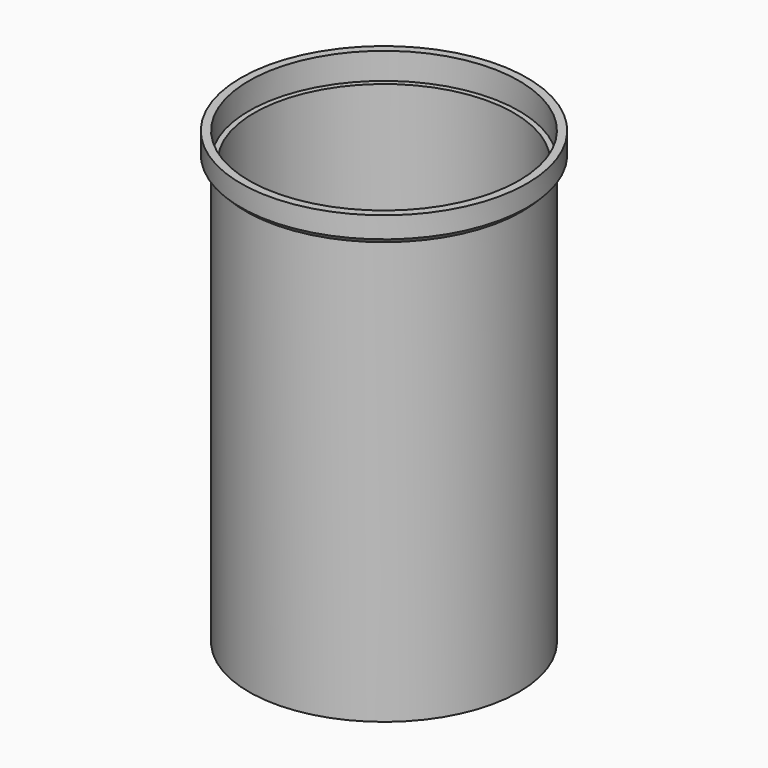
from build123d import *

# Parameters (mm, degrees)
F0_R          = 32.385
F1_DEPTH      = 101.6
F2_R          = 31.115
F3_DEPTH      = 99.06
F4_R          = 3.0308866689
F5_DEPTH      = 88.9
F5_DEPTH_BACK = 6.35
F6_R          = 34.3131351295
F6_R_2        = 32.385
F7_DEPTH      = 6.35
F8_SIZE       = 1.27


with BuildPart() as f1:
    # F0 (on Top) → F1 (new body)
    with BuildSketch(Plane.XY):
        Circle(F0_R)
    extrude(amount=F1_DEPTH)

    # F2 (on face) → F3 (cut)
    with BuildSketch(Plane.XY.offset(101.6)):
        Circle(F2_R)
    extrude(amount=-F3_DEPTH, mode=Mode.SUBTRACT)

    # F4 (on face) → F5 (cut, two sides)
    with BuildSketch(Plane.XY) as f5_sk:
        with Locations((-26.1913072318, 0)):
            Circle(F4_R)
        with Locations((-12.9833072318, 0)):
            Circle(F4_R)
        with Locations((0.2246927682, 0)):
            Circle(F4_R)
        with Locations((-21.1892126554, -15.3948641291)):
            Circle(F4_R)
        with Locations((-8.0935590395, -24.9094134131)):
            Circle(F4_R)
        with Locations((8.0935590395, -24.9094134131)):
            Circle(F4_R)
        with Locations((21.1892126554, -15.3948641291)):
            Circle(F4_R)
        with Locations((26.1913072318, 0)):
            Circle(F4_R)
        with Locations((21.1892126554, 15.3948641291)):
            Circle(F4_R)
        with Locations((8.0935590395, 24.9094134131)):
            Circle(F4_R)
        with Locations((-8.0935590395, 24.9094134131)):
            Circle(F4_R)
        with Locations((-21.1892126554, 15.3948641291)):
            Circle(F4_R)
        with Locations((-8.0949596534, -10.1507583404)):
            Circle(F4_R)
        with Locations((2.8890576511, -12.6577886127)):
            Circle(F4_R)
        with Locations((11.6975556182, -5.6332458878)):
            Circle(F4_R)
        with Locations((11.6975556182, 5.6332458878)):
            Circle(F4_R)
        with Locations((2.8890576511, 12.6577886127)):
            Circle(F4_R)
        with Locations((-8.0949596534, 10.1507583404)):
            Circle(F4_R)
    extrude(amount=-F5_DEPTH, mode=Mode.SUBTRACT)
    extrude(f5_sk.sketch, amount=F5_DEPTH_BACK, mode=Mode.SUBTRACT)


with BuildPart() as f7:
    # F6 (on face) → F7 (new body)
    with BuildSketch(Plane.XY.offset(101.6)):
        Circle(F6_R)
        Circle(F6_R_2, mode=Mode.SUBTRACT)
    extrude(amount=F7_DEPTH)

    # F8
    f8_edges = [f7.edges().sort_by_distance(p)[0] for p in [
        (-34.313135, 0, 101.6),
    ]]
    chamfer(f8_edges, length=F8_SIZE)


solid = Compound([f1.part, f7.part])
